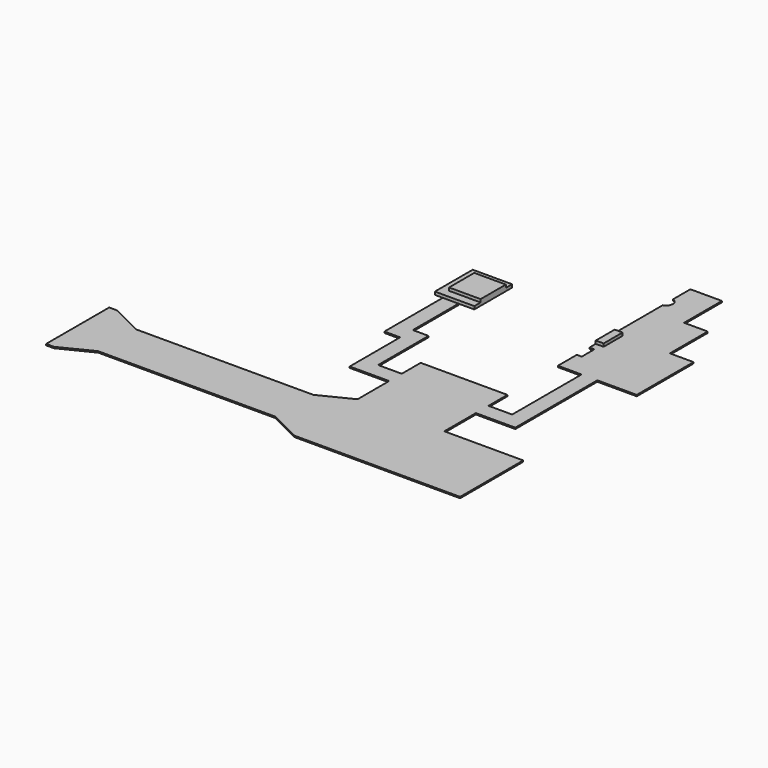
from build123d import *

# Parameters (mm, degrees)
F1_DEPTH = 100.584
F0_W     = 609.6
F0_H     = 1828.8
F2_DEPTH = 228.6
F0_W_2   = 2438.4
F0_H_2   = 2438.4
F3_DEPTH = 457.2


# Not quite as in the source:
# - a feature names something its author has since deleted; it is built from what else it names


with BuildPart() as f1:
    # F0 (on Top) → F1 (new body)
    with BuildSketch(Plane.XY):
        with BuildLine():
            Line((0, -1828.8), (0, 0))
            Line((0, 0), (-6705.6, 0))
            Line((-6705.6, 0), (-6705.6, -1828.8))
            Line((-6705.6, -1828.8), (-8534.4, -1828.8))
            Line((-8534.4, -1828.8), (-8534.4, 3048))
            Line((-8534.4, 3048), (-9753.6, 3048))
            Line((-9753.6, 3048), (-9753.6, 7467.6))
            Line((-9753.6, 7467.6), (-10972.8, 7467.6))
            Line((-10972.8, 7467.6), (-10972.8, 1828.8))
            Line((-10972.8, 1828.8), (-9753.6, 1828.8))
            Line((-9753.6, 1828.8), (-9753.6, -3048))
            Line((-9753.6, -3048), (-6705.6, -3048))
            Line((-6705.6, -3048), (-6705.6, -6096))
            Line((-6705.6, -6096), (-9144, -7315.2))
            Line((-9144, -7315.2), (-22860, -7315.2))
            Line((-22860, -7315.2), (-25298.4, -6096))
            Line((-25298.4, -6096), (-25908, -6096))
            Line((-25908, -6096), (-25908, -12192))
            Line((-25908, -12192), (-25298.4, -12192))
            Line((-25298.4, -12192), (-22860, -10972.8))
            Line((-22860, -10972.8), (-9144, -10972.8))
            Line((-9144, -10972.8), (-6705.6, -12192))
            Line((-6705.6, -12192), (6096, -12192))
            Line((6096, -12192), (6096, -6096))
            Line((6096, -6096), (0, -6096))
            Line((0, -6096), (0, -3048))
            Line((0, -3048), (3048, -3048))
            Line((3048, -3048), (3048, 4876.8))
            Line((3048, 4876.8), (4267.2, 4876.8))
            Line((4267.2, 4876.8), (6096, 4876.8))
            Line((6096, 4876.8), (6096, 10363.2))
            Line((6096, 10363.2), (4267.2, 10363.2))
            Line((4267.2, 10363.2), (4267.2, 14020.8))
            Line((4267.2, 14020.8), (2438.4, 14020.8))
            Line((2438.4, 14020.8), (2438.4, 17678.4))
            Line((2438.4, 17678.4000000001), (0, 17678.4000000001))
            Line((0, 17678.4), (0, 16002))
            ThreePointArc((0, 16002), (381, 15506.7), (0, 15011.4))
            Line((0, 15011.4), (0, 14020.8))
            Line((0, 14020.8), (457.2, 13106.4))
            Line((457.2, 13106.4), (457.2, 11277.6))
            Line((457.2, 11277.6), (0, 10363.2))
            Line((0, 10363.2), (609.6, 10363.2))
            Line((609.6, 10363.2), (609.6, 8534.4))
            Line((609.6, 8534.4), (0, 8534.4))
            Line((0, 8534.4), (0, 7924.8))
            Line((0, 7924.8), (381, 7924.8))
            Line((381, 7924.8), (381, 6705.6))
            Line((381, 6705.6), (0, 6705.6))
            Line((0, 6705.6), (0, 4876.8))
            Line((0, 4876.8), (1828.8, 4876.8))
            Line((1828.8, 4876.8), (1828.8, -1828.8))
            Line((1828.8, -1828.8), (0, -1828.8))
        make_face()
        Polygon((0, 14020.8), (0, 10363.2), (457.2, 11277.6), (457.2, 13106.4), align=None)
    extrude(amount=-F1_DEPTH)

    # F0 (on Top) → F2 (join)
    with BuildSketch(Plane.XY):
        with Locations((304.8, 9448.8)):
            Rectangle(F0_W, F0_H)
        Polygon((-10972.8, 7467.6), (-9753.6, 7467.6), (-8534.4, 7467.6), (-8534.4, 8077.2), (-10972.8, 8077.2), (-10972.8, 10515.6), (-8534.4, 10515.6), (-8534.4, 11125.2), (-11582.4, 11125.2), (-11582.4, 7467.6), align=None)
    extrude(amount=F2_DEPTH)

    # F0 (on Top) → F3 (join)
    with BuildSketch(Plane.XY):
        with Locations((-9753.6, 9296.4)):
            Rectangle(F0_W_2, F0_H_2)
    extrude(amount=F3_DEPTH)


solid = f1.part
